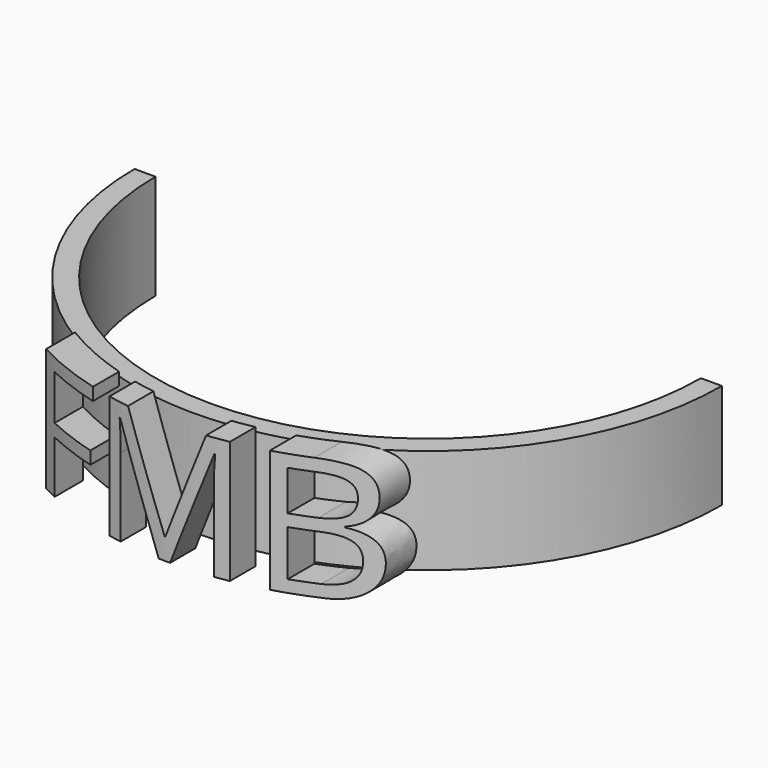
from build123d import *

# Parameters (mm, degrees)
F0_TEXT_SIZE = 20.7939804364
F1_DEPTH     = 32.512
F3_START     = -22.86
F3_DEPTH     = 35.052
F5_DEPTH     = 12.7


# Not quite as in the source:
# - Text() gives the source's letters only with a copy of the font that has no kerning and outlines rounded to 1/6400 em; it was checked with that copy


with BuildPart() as f1:
    # F0 (on Front) → F1 (new body)
    with BuildSketch(Plane.XZ):
        with Locations((-5.2083201593, -14.3467716174)):
            Text('FMB', F0_TEXT_SIZE, font='Open Sans', text_align=(TextAlign.LEFT, TextAlign.BOTTOM))
    extrude(amount=F1_DEPTH)

    # F2 (on Top) → F3 (intersect)
    with BuildSketch(Plane.XY.offset(F3_START)):
        with BuildLine():
            ThreePointArc((50.8488743876, 12.7), (15.2888743876, -22.86), (-20.2711256124, 12.7))
            Line((-20.2711256124, 12.7), (-24.0811256124, 12.7))
            ThreePointArc((-24.0811256124, 12.7), (15.2888743876, -26.67), (54.6588743876, 12.7))
            Line((54.6588743876, 12.7), (50.8488743876, 12.7))
        make_face()
    extrude(amount=F3_DEPTH, mode=Mode.INTERSECT)

    # F4 (on Top) → F5 (join)
    with BuildSketch(Plane.XY):
        with BuildLine():
            ThreePointArc((-20.2711256124, 12.7), (15.2888743876, -22.86), (50.8488743876, 12.7))
            Line((50.8488743876, 12.7), (48.3088743876, 12.7))
            ThreePointArc((48.3088743876, 12.7), (15.2888743876, -20.32), (-17.7311256124, 12.7))
            Line((-17.7311256124, 12.7), (-20.2711256124, 12.7))
        make_face()
    extrude(amount=-F5_DEPTH)


solid = f1.part
